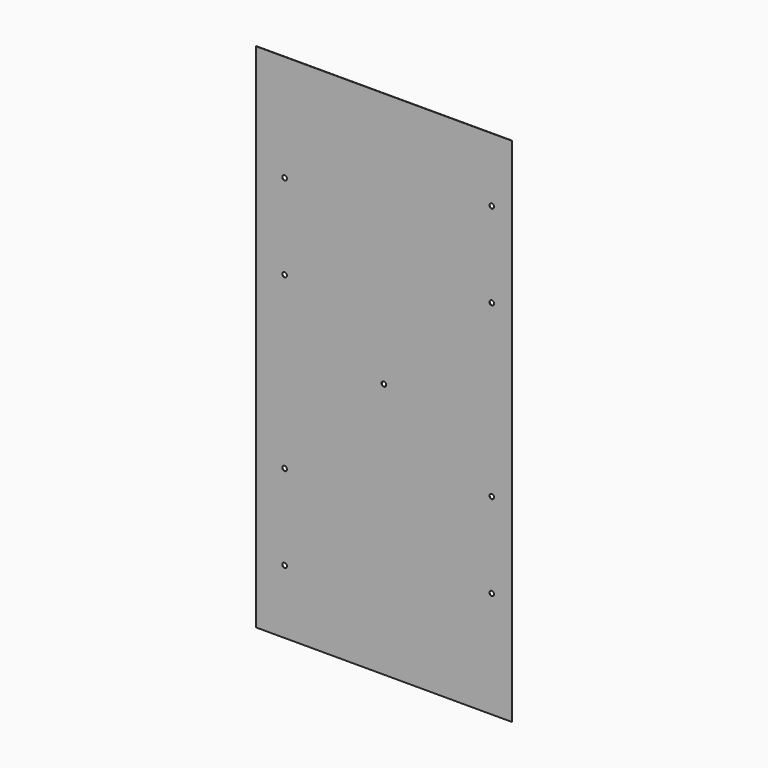
from build123d import *

# Parameters (mm, degrees)
F0_W     = 609.6
F0_H     = 1219.2
F1_DEPTH = 0.79375
F2_R     = 5.55625
F3_DEPTH = 25.4
F4_R     = 5.55625
F5_DEPTH = 25.4


# Not quite as in the source:
# - a feature names something its author has since deleted; it is built from what else it names


with BuildPart() as f1:
    # F0 (on Front) → F1 (new body)
    with BuildSketch(Plane.XZ):
        with Locations((304.8, 609.6)):
            Rectangle(F0_W, F0_H)
    extrude(amount=F1_DEPTH)

    # F2 (on face) → F3 (cut)
    with BuildSketch(Plane.XZ.offset(0.79375)):
        with Locations((68.2625, 152.4)):
            Circle(F2_R)
        with Locations((68.2625, 355.6)):
            Circle(F2_R)
        with Locations((561.975, 863.6)):
            Circle(F2_R)
        with Locations((561.975, 1066.8)):
            Circle(F2_R)
        with Locations((561.975, 254)):
            Circle(F2_R)
        with Locations((561.975, 457.2)):
            Circle(F2_R)
        with Locations((68.2625, 762)):
            Circle(F2_R)
        with Locations((68.2625, 965.2)):
            Circle(F2_R)
    extrude(amount=-F3_DEPTH, mode=Mode.SUBTRACT)

    # F4 (on face) → F5 (cut)
    with BuildSketch(Plane.XZ.offset(0.79375)):
        with Locations((304.8, 609.6)):
            Circle(F4_R)
    extrude(amount=-F5_DEPTH, mode=Mode.SUBTRACT)


solid = f1.part
